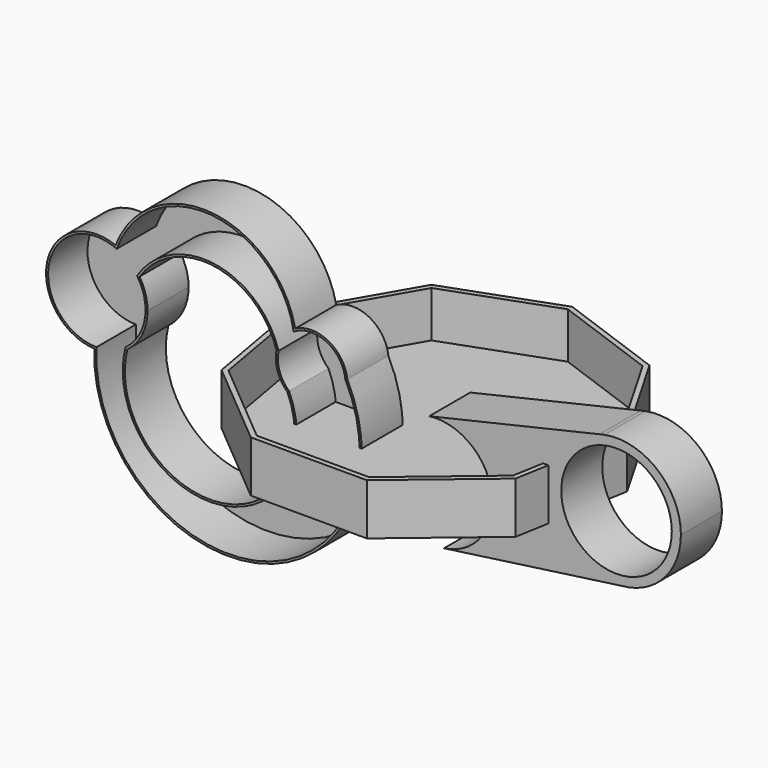
from build123d import *

# Parameters (mm, degrees)
F0_R     = 26.9464960859
F1_DEPTH = 25
F3_DEPTH = 25
F4_T     = -1
F6_DEPTH = 25
F7_T     = -2.5


# Not quite as in the source:
# - a feature of the source that left no trace in its solid (it failed there, or was rolled back) is left out
# - the program builds the solid bodies; features that only make, move or delete a surface that nothing else refers to are left out


with BuildPart() as f1:
    # F0 (on Front) → F1 (new body)
    with BuildSketch(Plane.XZ):
        with BuildLine():
            Line((40.761068845, 47.0056567036), (38.2815639413, 46.4308663652))
            ThreePointArc((38.2815639413, 46.4308663652), (15.703663518, 10.6659749386), (49.2399074327, -15.1062851558))
            Line((49.2399074327, -15.1062851558), (52.5844195802, -14.6420472673))
            ThreePointArc((52.5844195802, -14.6420472673), (70.8188113885, -3.7982421999), (77.988971946, 16.1684788764))
            ThreePointArc((77.988971946, 16.1684788764), (66.6245182731, 40.3389583174), (40.761068845, 47.0056567036))
        make_face()
        with Locations((46.6032624245, 16.1684788764)):
            Circle(F0_R, mode=Mode.SUBTRACT)
        with BuildLine():
            ThreePointArc((-44.7106001415, 27.1919070038), (-23.151428053, 20.5583413445), (-13.8693649386, 0))
            ThreePointArc((-13.8693649386, 0), (-20.6075462255, -17.9987370156), (-37.5089408348, -27.1475337383))
            Line((-37.5089408348, -27.1475337383), (49.2399074327, -15.1062851558))
            ThreePointArc((49.2399074327, -15.1062851558), (15.703663518, 10.6659749386), (38.2815639413, 46.4308663652))
            Line((38.2815639413, 46.4308663652), (-44.7106001415, 27.1919070038))
        make_face()
    extrude(amount=F1_DEPTH)


with BuildPart() as f3:
    # F2 (on Front) → F3 (new body)
    with BuildSketch(Plane.XZ):
        with BuildLine():
            ThreePointArc((-197.6164360222, 50.8064648047), (-230.9491852504, 33.0606563326), (-207.9779482368, 3.0888669381))
            ThreePointArc((-207.9779482368, 3.0888669381), (-199.5168720301, 4.1435435485), (-191.9158228131, 8.0069881422))
            ThreePointArc((-191.9158228131, 8.0069881422), (-184.626891673, 16.7388855513), (-182.0132419339, 27.8088171035))
            ThreePointArc((-182.0132419339, 27.8088171035), (-183.0104691396, 34.7635176788), (-185.921789492, 41.1577757279))
            ThreePointArc((-185.921789492, 41.1577757279), (-191.012098095, 46.8996561949), (-197.6164360222, 50.8064648047))
        make_face()
        with BuildLine():
            ThreePointArc((-119.2122107169, 31.2843508649), (-116.0438313369, 38.4743002747), (-110.0490633826, 43.5533511295))
            ThreePointArc((-110.0490633826, 43.5533511295), (-151.1091973781, 80.0615546597), (-197.6164360222, 50.8064648047))
            ThreePointArc((-197.6164360222, 50.8064648047), (-191.012098095, 46.8996561949), (-185.921789492, 41.1577757279))
            ThreePointArc((-185.921789492, 41.1577757279), (-149.4196390648, 57.4861392064), (-119.2122107169, 31.2843508649))
        make_face()
        with BuildLine():
            ThreePointArc((-113.8456945473, 15.100368808), (-94.9747299387, 11.984555216), (-84.5226842358, 28.0025557225))
            ThreePointArc((-84.5226842358, 28.0025557225), (-84.552889755, 29.030310945), (-84.6434020412, 30.0545182956))
            ThreePointArc((-84.6434020412, 30.0545182956), (-93.811483299, 43.4565577664), (-110.0490633826, 43.5533511295))
            ThreePointArc((-110.0490633826, 43.5533511295), (-116.0438313369, 38.4743002747), (-119.2122107169, 31.2843508649))
            ThreePointArc((-119.2122107169, 31.2843508649), (-118.6332875237, 22.4945743852), (-113.8456945473, 15.100368808))
        make_face()
        with BuildLine():
            ThreePointArc((-84.6434020412, 30.0545182956), (-84.552889755, 29.030310945), (-84.5226842358, 28.0025557225))
            ThreePointArc((-84.5226842358, 28.0025557225), (-94.9747299387, 11.984555216), (-113.8456945473, 15.100368808))
            ThreePointArc((-113.8456945473, 15.100368808), (-147.9079885613, -43.1768963111), (-191.9158228131, 8.0069881422))
            ThreePointArc((-191.9158228131, 8.0069881422), (-199.5168720301, 4.1435435485), (-207.9779482368, 3.0888669381))
            ThreePointArc((-207.9779482368, 3.0888669381), (-128.8530958523, -63.275168505), (-84.6434020412, 30.0545182956))
        make_face()
    extrude(amount=F3_DEPTH)

    # F4
    f4_openings = [f3.faces().sort_by_distance(p)[0] for p in [
        (-228.882394, -25, 32.611868),
    ]]
    offset(amount=F4_T, openings=f4_openings, kind=Kind.INTERSECTION)


with BuildPart() as f6:
    # F5 (on Top) → F6 (new body)
    with BuildSketch(Plane.XY):
        Polygon((-89.5143109171, -77.751763165), (-32.9156560095, -77.751763165), (10.4414290704, -41.3708490655), (20.2696823535, 14.3679450975), (-8.0296451003, 63.3838180675), (-61.2149834633, 82.741698131), (-114.4003218263, 63.3838180675), (-142.6996492801, 14.3679450975), (-132.871395997, -41.3708490655), align=None)
    extrude(amount=F6_DEPTH)

    # F7
    f7_openings = [f6.faces().sort_by_distance(p)[0] for p in [
        (-61.214983, 0, 25),
    ]]
    offset(amount=F7_T, openings=f7_openings)


solid = Compound([f1.part, f3.part, f6.part])
